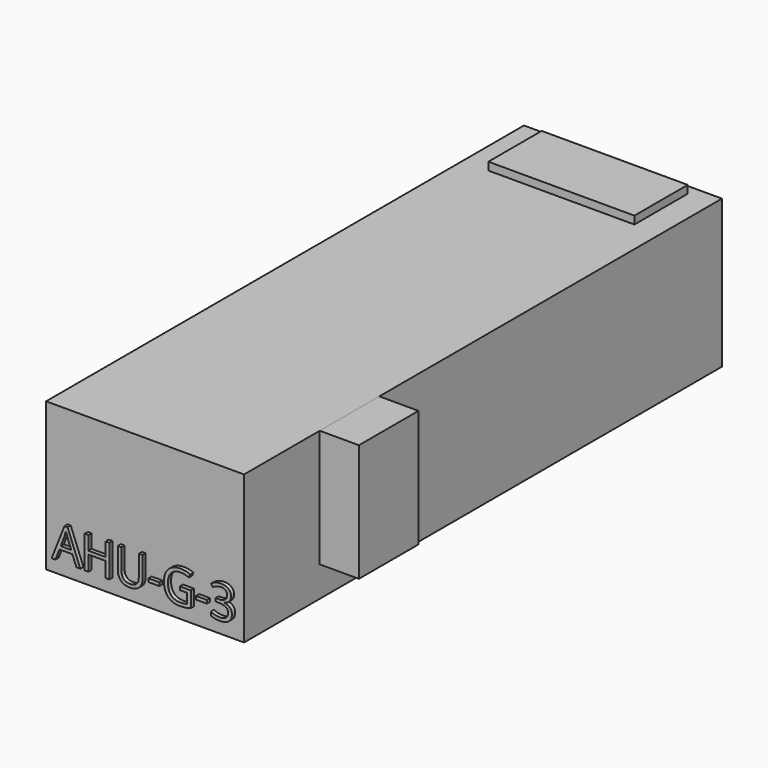
from build123d import *

# Parameters (mm, degrees)
F0_W         = 1282.7
F0_H         = 958.85
F1_DEPTH     = 3870.325
F2_W         = 482.6
F2_H         = 482.6
F3_DEPTH     = 50.8
F4_W         = 482.6
F4_H         = 762
F5_DEPTH     = 254
F6_TEXT_SIZE = 293.2465117839
F7_DEPTH     = 25.4
F8_W         = 946.15
F8_H         = 431.8
F9_DEPTH     = 50.8
F10_W        = 946.15
F10_H        = 431.8
F11_DEPTH    = 50.8


# Not quite as in the source:
# - Text() gives the source's letters only with a copy of the font that has no kerning and outlines rounded to 1/6400 em; it was checked with that copy


with BuildPart() as f1:
    # F0 (on Front) → F1 (new body)
    with BuildSketch(Plane.XZ):
        with Locations((1.4098696411, -73.0132179465)):
            Rectangle(F0_W, F0_H)
    extrude(amount=F1_DEPTH)

    # F2 (on face) → F3 (join)
    with BuildSketch(Plane(origin=(-639.9401303589, 0, 0), x_dir=(0, -1, 0), z_dir=(-1, 0, 0))):
        with Locations((3521.075, 50.8117820535)):
            Rectangle(F2_W, F2_H)
    extrude(amount=F3_DEPTH)

    # F6 (on face) → F7 (join)
    with BuildSketch(Plane.XZ.offset(3870.325)):
        with Locations((-583.5361480713, -459.9448442459)):
            Text('AHU-G-3', F6_TEXT_SIZE, font='Open Sans', text_align=(TextAlign.LEFT, TextAlign.BOTTOM))
    extrude(amount=F7_DEPTH)

    # F8 (on face) → F9 (join)
    with BuildSketch(Plane.XY.offset(406.4117820535)):
        with Locations((1.4098696411, -282.575)):
            Rectangle(F8_W, F8_H)
    extrude(amount=F9_DEPTH)

    # F10 (on face) → F11 (join)
    with BuildSketch(Plane(origin=(0, 0, 0), x_dir=(-1, 0, 0), z_dir=(0, 1, 0))):
        with Locations((-1.4098696411, -38.0882179465)):
            Rectangle(F10_W, F10_H)
    extrude(amount=F11_DEPTH)


with BuildPart() as f5:
    # F4 (on face) → F5 (new body)
    with BuildSketch(Plane.YZ.offset(642.7598696411)):
        with Locations((-3016.25, 25.4117820535)):
            Rectangle(F4_W, F4_H)
    extrude(amount=F5_DEPTH)


solid = Compound([f1.part, f5.part])
